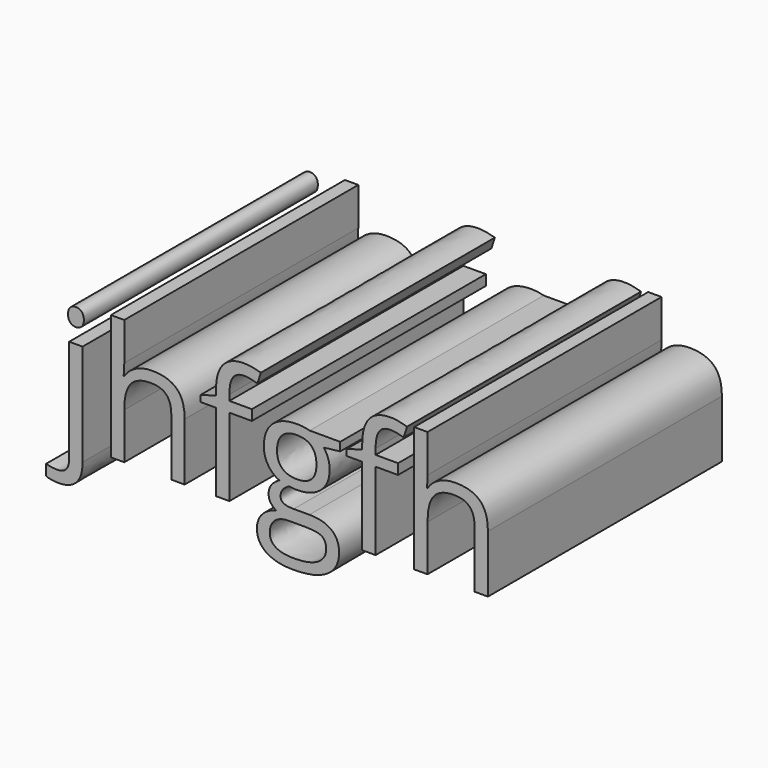
from build123d import *

# Parameters (mm, degrees)
F0_TEXT_SIZE = 14.3177134709
F1_DEPTH     = 25.4


# Not quite as in the source:
# - Text() gives the source's letters only with a copy of the font that has no kerning and outlines rounded to 1/6400 em; it was checked with that copy


with BuildPart() as f1:
    # F0 (on Front) → F1 (new body)
    with BuildSketch(Plane.XZ):
        with Locations((-66.5383338928, 54.0038235486)):
            Text('jhfgfh', F0_TEXT_SIZE, font='Open Sans', text_align=(TextAlign.LEFT, TextAlign.BOTTOM))
    extrude(amount=F1_DEPTH)


solid = f1.part
